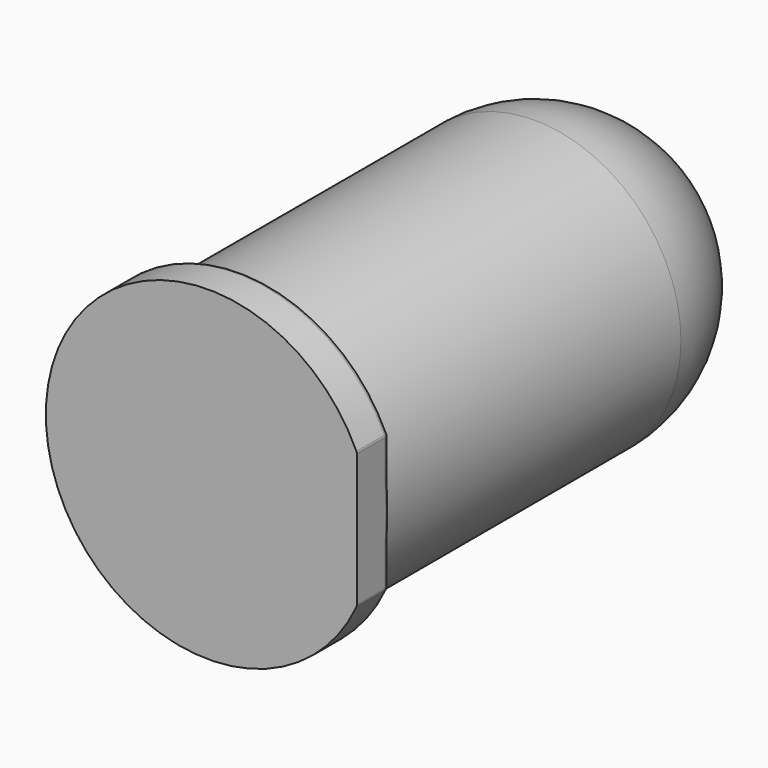
from build123d import *

# Parameters (mm, degrees)
F2_W     = 0.225
F2_H     = 0.6141559725
F3_DEPTH = 12.5
F4_R     = 0.075


with BuildPart() as f1:
    # F0 (on Top) → F1 (revolve)
    with BuildSketch(Plane.XY):
        with BuildLine():
            Line((-101.5040925145, -14.4654285704), (-101.5040925145, -9.9654285704))
            ThreePointArc((-101.5040925145, -9.9654285704), (-103.0950827722, -10.6244383127), (-103.7540925145, -12.2154285704))
            ThreePointArc((-103.7540925145, -12.2154285704), (-103.0950827722, -13.8064188281), (-101.5040925145, -14.4654285704))
        make_face()
        with BuildLine():
            Line((-101.5040925145, -17.8512725979), (-101.5040925145, -14.4654285704))
            ThreePointArc((-101.5040925145, -14.4654285704), (-103.0950827722, -13.8064188281), (-103.7540925145, -12.2154285704))
            Line((-103.7540925145, -12.2154285704), (-103.7540925145, -17.8512725979))
            Line((-103.7540925145, -17.8512725979), (-101.5040925145, -17.8512725979))
        make_face()
        Polygon((-101.5040925145, -18.4654285704), (-101.5040925145, -17.8512725979), (-103.7540925145, -17.8512725979), (-104.0040925145, -17.8512725979), (-104.0040925145, -18.4654285704), align=None)
    revolve(axis=Axis((-101.5040925145, -14.2154285704, 0), (0, -1, 0)))

    # F2 (on Top) → F3 (cut, symmetric)
    with BuildSketch(Plane.XY):
        with Locations((-99.1165925145, -18.1583505842)):
            Rectangle(F2_W, F2_H)
    extrude(amount=F3_DEPTH, both=True, mode=Mode.SUBTRACT)

    # F4
    f4_edges = [f1.edges().sort_by_distance(p)[0] for p in [
        (-104.004093, -17.851273, 0),
        (-99.229093, -17.851273, 0),
        (-99.229093, -18.158351, 1.036521),
        (-99.229093, -18.158351, -1.036521),
    ]]
    fillet(f4_edges, radius=F4_R)


solid = f1.part
